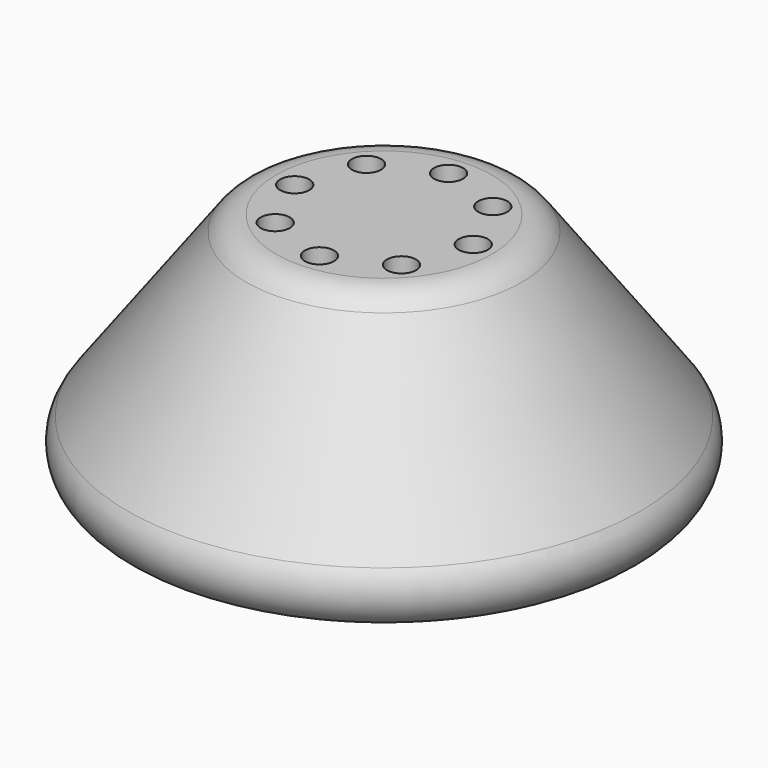
from build123d import *

# Parameters (mm, degrees)
F2_R            = 5.08
F3_R            = 2.006915686
F4_DEPTH        = 25.4
F4_COPIES_COUNT = 8


# Not quite as in the source:
# - a pattern or mirror of a feature is missing from the dataset's text; its kind, count and spacing are read off the source's solid


with BuildPart() as f1:
    # F0 (on Front) → F1 (revolve)
    with BuildSketch(Plane.XZ):
        Polygon((0, 23.1683626771), (0, 55.6904152036), (-17.4122489989, 55.6904152036), (-41.3001254201, 23.1683626771), align=None)
    revolve(axis=Axis((0, 0, 39.4293889403), (0, 0, 1)))

    # F2
    f2_edges = [f1.edges().sort_by_distance(p)[0] for p in [
        (41.300125, 0, 23.168363),
        (17.412249, 0, 55.690415),
    ]]
    fillet(f2_edges, radius=F2_R)

    # F3 (on face) → F4 (cut)
    with BuildSketch(Plane.XY.offset(55.6904152036)):
        with Locations((-8.7765334174, 7.9615563154)):
            Circle(F3_R)
    f4 = extrude(amount=-F4_DEPTH, mode=Mode.SUBTRACT)

    # F4_copies: F4 ×8 about axis
    f4_copies_axis = Axis((0, 0, 0), (0, 0, 1))
    for i in range(1, F4_COPIES_COUNT):
        add(f4.rotate(f4_copies_axis, i * 360 / F4_COPIES_COUNT), mode=Mode.SUBTRACT)


solid = f1.part
